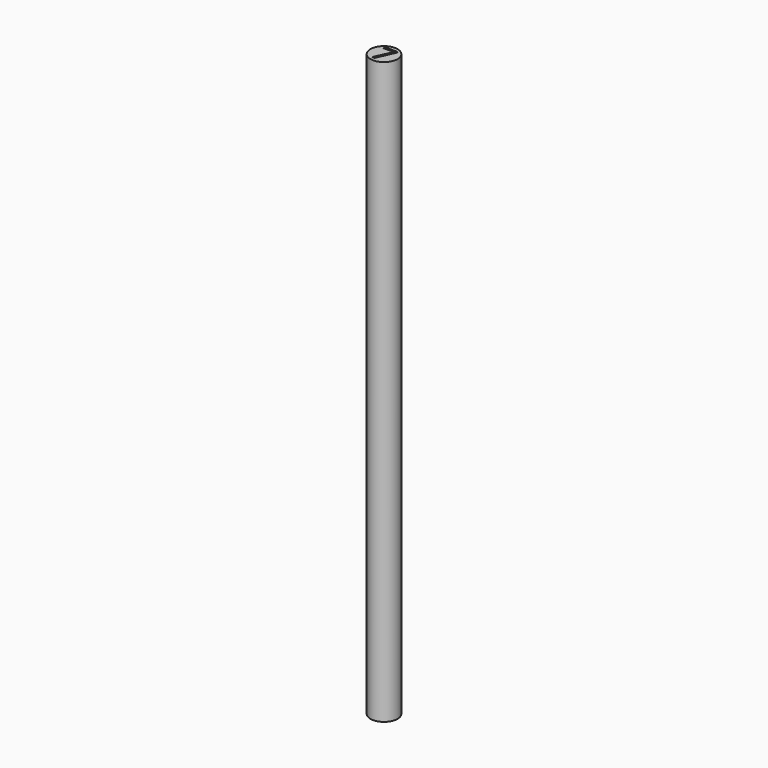
from build123d import *

# Parameters (mm, degrees)
F0_R         = 3.5
F1_DEPTH     = 150
F2_TEXT_SIZE = 6.9444444444
F3_DEPTH     = 1
F4_TEXT_SIZE = 6.9444444444
F5_DEPTH     = 1


# Not quite as in the source:
# - Text() gives the source's letters only with a copy of the font that has no kerning and outlines rounded to 1/6400 em; it was checked with that copy


with BuildPart() as f1:
    # F0 (on Top) → F1 (new body)
    with BuildSketch(Plane.XY):
        Circle(F0_R)
    extrude(amount=F1_DEPTH)

    # F2 (on face) → F3 (cut)
    with BuildSketch(Plane(origin=(0, 0, 0), x_dir=(1, 0, 0), z_dir=(0, 0, -1))):
        with Locations((-2.0339626736, -2.5)):
            Text('7', F2_TEXT_SIZE, font='Open Sans', text_align=(TextAlign.LEFT, TextAlign.BOTTOM))
    extrude(amount=-F3_DEPTH, mode=Mode.SUBTRACT)

    # F4 (on face) → F5 (cut)
    with BuildSketch(Plane.XY.offset(150)):
        with Locations((-2.0339626736, -2.5)):
            Text('7', F4_TEXT_SIZE, font='Open Sans', text_align=(TextAlign.LEFT, TextAlign.BOTTOM))
    extrude(amount=-F5_DEPTH, mode=Mode.SUBTRACT)


solid = f1.part
